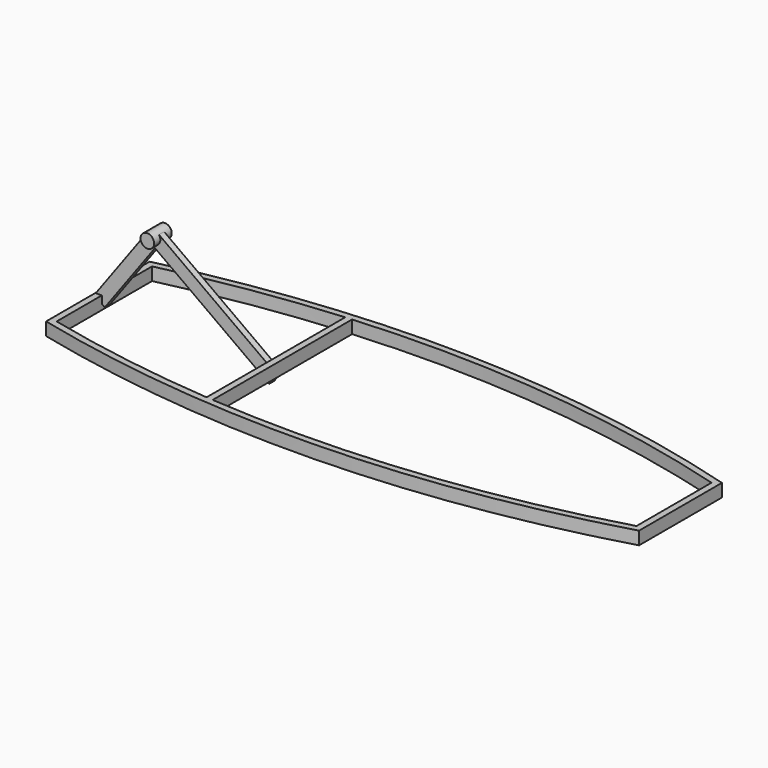
from build123d import *

# Parameters (mm, degrees)
F1_DEPTH = 40
F3_R     = 21
F4_DEPTH = 34
F6_DEPTH = 10
F8_DEPTH = 10


with BuildPart() as f1:
    # F0 (on Top) → F1 (new body)
    with BuildSketch(Plane.XY):
        with BuildLine():
            Line((1800, 0), (1800, 160))
            ThreePointArc((1800, 160), (902.6160702853, 297.723162839), (0, 200))
            Line((0, 200), (0, 0))
            Line((0, 0), (20, 0))
            Line((20, 0), (20, 184.2338650593))
            ThreePointArc((20, 184.2338650593), (283.3887356677, 236.2041785507), (550, 267.7156572871))
            Line((550, 267.7156572871), (550, 0))
            Line((550, 0), (570, 0))
            Line((570, 0), (570, 269.2422609738))
            ThreePointArc((570, 269.2422609738), (1180.4728881109, 260.3694842678), (1780, 144.9436838818))
            Line((1780, 144.9436838818), (1780, 0))
            Line((1780, 0), (1800, 0))
        make_face()
    extrude(amount=F1_DEPTH)

    # F2: F1 across plane


with BuildPart() as f1_1:
    add(f1.part)
    add(f1.part.mirror(Plane.XZ))


with BuildPart() as f4:
    # F3 (on Front) → F4 (new body, symmetric)
    with BuildSketch(Plane.XZ):
        with Locations((180, 250)):
            Circle(F3_R)
    extrude(amount=F4_DEPTH, both=True)

    # F5 (on Front) → F6 (join, symmetric)
    with BuildSketch(Plane.XZ):
        Polygon((196.1360515255, 238.1835774803), (163.8639484745, 261.8164225197), (-2.9672317155, 33.9981877608), (29.3048713356, 10.3653427213), align=None)
    extrude(amount=F6_DEPTH, both=True)


with BuildPart() as f8:
    # F7 (on Front) → F8 (new body, symmetric)
    with BuildSketch(Plane.XZ):
        Polygon((560.4952573776, 0), (191.7060117653, 266.216327838), (180, 250), (548.7892456123, -16.216327838), align=None)
        Polygon((548.7892456123, -16.216327838), (180, 250), (168.2939882347, 233.783672162), (537.083233847, -32.4326556761), align=None)
    extrude(amount=F8_DEPTH, both=True)


solid = Compound([f1_1.part, f4.part, f8.part])
